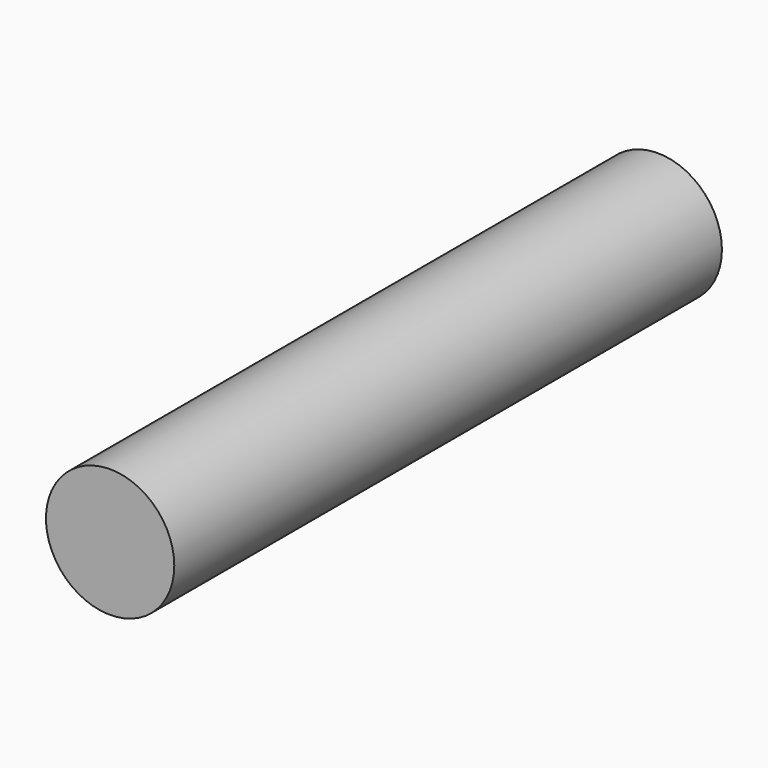
from build123d import *

# Parameters (mm, degrees)
F0_R          = 47.6123806479
F1_DEPTH      = 254
F1_DEPTH_BACK = 254


# Not quite as in the source:
# - the program builds the solid bodies; features that only make, move or delete a surface that nothing else refers to are left out


with BuildPart() as f1:
    # F0 (on Front) → F1 (new body, two sides)
    with BuildSketch(Plane.XZ) as f1_sk:
        Circle(F0_R)
    extrude(amount=F1_DEPTH)
    extrude(f1_sk.sketch, amount=-F1_DEPTH_BACK)


solid = f1.part
